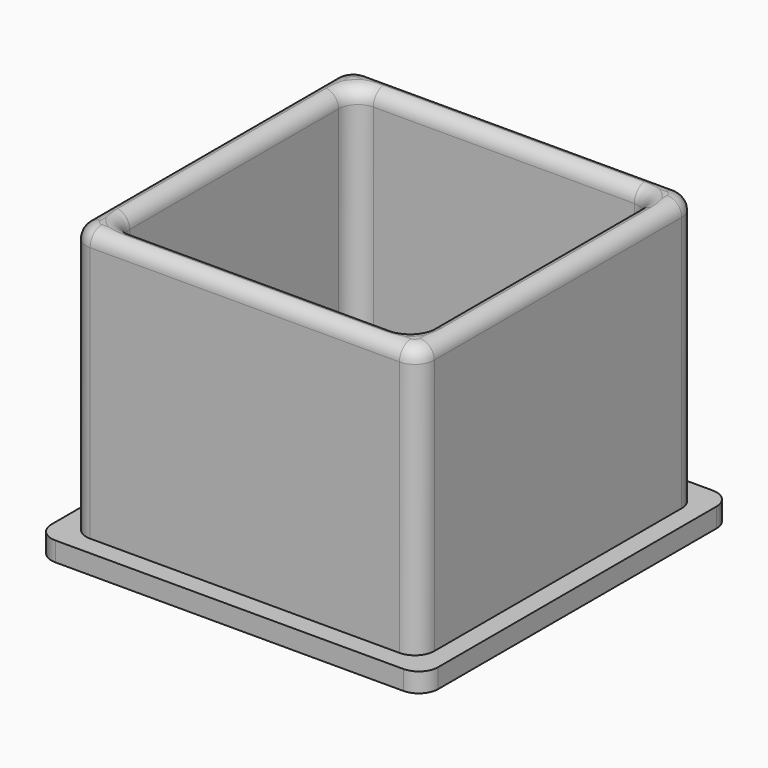
from build123d import *

# Parameters (mm, degrees)
F0_W         = 36
F0_H         = 36
F1_DEPTH     = 2
F2_DEPTH     = 30
F3_T         = -2.5
F4_R         = 2
F5_T1_DEPTH  = 32
F5_T3_DEPTH  = 27
F5_T5_DEPTH  = 32
F5_T7_DEPTH  = 27
F5_T10_ANGLE = 90
F5_T12_ANGLE = 90
F5_T14_ANGLE = 90
F5_T16_ANGLE = 90
F5_T18_ANGLE = 90
F5_T20_ANGLE = 90
F5_T22_ANGLE = 90
F5_T24_ANGLE = 90


# Not quite as in the source:
# - a fillet or chamfer that OpenCascade refuses, or shapes differently, is made with other operations: its cross-section is extruded or revolved along the edge and cut away or added


with BuildPart() as f1:
    # F0 (on Top) → F1 (new body)
    with BuildSketch(Plane.XY):
        with BuildLine():
            ThreePointArc((20, 18), (19.4142135624, 19.4142135624), (18, 20))
            Line((18, 20), (-18, 20))
            ThreePointArc((-18, 20), (-19.4142135624, 19.4142135624), (-20, 18))
            Line((-20, 18), (-20, -18))
            ThreePointArc((-20, -18), (-19.4142135624, -19.4142135624), (-18, -20))
            Line((-18, -20), (18, -20))
            ThreePointArc((18, -20), (19.4142135624, -19.4142135624), (20, -18))
            Line((20, -18), (20, 18))
        make_face()
        Rectangle(F0_W, F0_H, mode=Mode.SUBTRACT)
    extrude(amount=F1_DEPTH)

    # F0 (on Top) → F2 (join)
    with BuildSketch(Plane.XY):
        Rectangle(F0_W, F0_H)
    extrude(amount=F2_DEPTH)

    # F3
    f3_openings = [f1.faces().sort_by_distance(p)[0] for p in [
        (0, 0, 30),
    ]]
    offset(amount=F3_T, openings=f3_openings)

    # F4
    f4_edges = [f1.edges().sort_by_distance(p)[0] for p in [
        (-18, -18, 16),
        (18, 18, 16),
        (-18, 18, 16),
        (18, -18, 16),
        (-15.5, -15.5, 16.25),
        (15.5, -15.5, 16.25),
        (15.5, 15.5, 16.25),
        (-15.5, 15.5, 16.25),
    ]]
    fillet(f4_edges, radius=F4_R)

    # F5: fillet of radius 1.5 on 16 edges, made by hand

    # F5_s2 → F5_t1 (cut)
    with BuildSketch(Plane.XZ.offset(-16)):
        with BuildLine():
            ThreePointArc((-18, 28.5), (-17.5606601718, 29.5606601718), (-16.5, 30))
            Line((-16.5, 30), (-18, 30))
            Line((-18, 30), (-18, 28.5))
        make_face()
        with BuildLine():
            ThreePointArc((18, 28.5), (17.5606601718, 29.5606601718), (16.5, 30))
            Line((16.5, 30), (18, 30))
            Line((18, 30), (18, 28.5))
        make_face()
    extrude(amount=F5_T1_DEPTH, mode=Mode.SUBTRACT)

    # F5_s4 → F5_t3 (cut)
    with BuildSketch(Plane.XZ.offset(-13.5)):
        with BuildLine():
            ThreePointArc((-17, 30), (-15.9393398282, 29.5606601718), (-15.5, 28.5))
            Line((-15.5, 28.5), (-15.5, 30))
            Line((-15.5, 30), (-17, 30))
        make_face()
        with BuildLine():
            ThreePointArc((17, 30), (15.9393398282, 29.5606601718), (15.5, 28.5))
            Line((15.5, 28.5), (15.5, 30))
            Line((15.5, 30), (17, 30))
        make_face()
    extrude(amount=F5_T3_DEPTH, mode=Mode.SUBTRACT)

    # F5_s6 → F5_t5 (cut)
    with BuildSketch(Plane.YZ.offset(-16)):
        with BuildLine():
            ThreePointArc((18, 28.5), (17.5606601718, 29.5606601718), (16.5, 30))
            Line((16.5, 30), (18, 30))
            Line((18, 30), (18, 28.5))
        make_face()
        with BuildLine():
            ThreePointArc((-18, 28.5), (-17.5606601718, 29.5606601718), (-16.5, 30))
            Line((-16.5, 30), (-18, 30))
            Line((-18, 30), (-18, 28.5))
        make_face()
    extrude(amount=F5_T5_DEPTH, mode=Mode.SUBTRACT)

    # F5_s8 → F5_t7 (cut)
    with BuildSketch(Plane.YZ.offset(-13.5)):
        with BuildLine():
            ThreePointArc((-17, 30), (-15.9393398282, 29.5606601718), (-15.5, 28.5))
            Line((-15.5, 28.5), (-15.5, 30))
            Line((-15.5, 30), (-17, 30))
        make_face()
        with BuildLine():
            ThreePointArc((17, 30), (15.9393398282, 29.5606601718), (15.5, 28.5))
            Line((15.5, 28.5), (15.5, 30))
            Line((15.5, 30), (17, 30))
        make_face()
    extrude(amount=F5_T7_DEPTH, mode=Mode.SUBTRACT)

    # F5_s9 → F5_t10 (revolve, cut)
    with BuildSketch(Plane.YZ.offset(-16)):
        with BuildLine():
            ThreePointArc((18, 28.5), (17.5606601718, 29.5606601718), (16.5, 30))
            Line((16.5, 30), (18, 30))
            Line((18, 30), (18, 28.5))
        make_face()
    revolve(axis=Axis((-16, 16, 30), (0, 0, 1)), revolution_arc=F5_T10_ANGLE, mode=Mode.SUBTRACT)

    # F5_s11 → F5_t12 (revolve, cut)
    with BuildSketch(Plane.YZ.offset(16)):
        with BuildLine():
            ThreePointArc((18, 28.5), (17.5606601718, 29.5606601718), (16.5, 30))
            Line((16.5, 30), (18, 30))
            Line((18, 30), (18, 28.5))
        make_face()
    revolve(axis=Axis((16, 16, 30), (0, 0, -1)), revolution_arc=F5_T12_ANGLE, mode=Mode.SUBTRACT)

    # F5_s13 → F5_t14 (revolve, cut)
    with BuildSketch(Plane.YZ.offset(-16)):
        with BuildLine():
            ThreePointArc((-18, 28.5), (-17.5606601718, 29.5606601718), (-16.5, 30))
            Line((-16.5, 30), (-18, 30))
            Line((-18, 30), (-18, 28.5))
        make_face()
    revolve(axis=Axis((-16, -16, 30), (0, 0, -1)), revolution_arc=F5_T14_ANGLE, mode=Mode.SUBTRACT)

    # F5_s15 → F5_t16 (revolve, cut)
    with BuildSketch(Plane.XZ.offset(16)):
        with BuildLine():
            ThreePointArc((18, 28.5), (17.5606601718, 29.5606601718), (16.5, 30))
            Line((16.5, 30), (18, 30))
            Line((18, 30), (18, 28.5))
        make_face()
    revolve(axis=Axis((16, -16, 30), (0, 0, -1)), revolution_arc=F5_T16_ANGLE, mode=Mode.SUBTRACT)

    # F5_s17 → F5_t18 (revolve, cut)
    with BuildSketch(Plane.XZ.offset(13.5)):
        with BuildLine():
            ThreePointArc((17, 30), (15.9393398282, 29.5606601718), (15.5, 28.5))
            Line((15.5, 28.5), (15.5, 30))
            Line((15.5, 30), (17, 30))
        make_face()
    revolve(axis=Axis((13.5, -13.5, 30), (0, 0, -1)), revolution_arc=F5_T18_ANGLE, mode=Mode.SUBTRACT)

    # F5_s19 → F5_t20 (revolve, cut)
    with BuildSketch(Plane.XZ.offset(-13.5)):
        with BuildLine():
            ThreePointArc((17, 30), (15.9393398282, 29.5606601718), (15.5, 28.5))
            Line((15.5, 28.5), (15.5, 30))
            Line((15.5, 30), (17, 30))
        make_face()
    revolve(axis=Axis((13.5, 13.5, 30), (0, 0, 1)), revolution_arc=F5_T20_ANGLE, mode=Mode.SUBTRACT)

    # F5_s21 → F5_t22 (revolve, cut)
    with BuildSketch(Plane.XZ.offset(13.5)):
        with BuildLine():
            ThreePointArc((-17, 30), (-15.9393398282, 29.5606601718), (-15.5, 28.5))
            Line((-15.5, 28.5), (-15.5, 30))
            Line((-15.5, 30), (-17, 30))
        make_face()
    revolve(axis=Axis((-13.5, -13.5, 30), (0, 0, 1)), revolution_arc=F5_T22_ANGLE, mode=Mode.SUBTRACT)

    # F5_s23 → F5_t24 (revolve, cut)
    with BuildSketch(Plane.YZ.offset(-13.5)):
        with BuildLine():
            ThreePointArc((17, 30), (15.9393398282, 29.5606601718), (15.5, 28.5))
            Line((15.5, 28.5), (15.5, 30))
            Line((15.5, 30), (17, 30))
        make_face()
    revolve(axis=Axis((-13.5, 13.5, 30), (0, 0, 1)), revolution_arc=F5_T24_ANGLE, mode=Mode.SUBTRACT)


solid = f1.part
